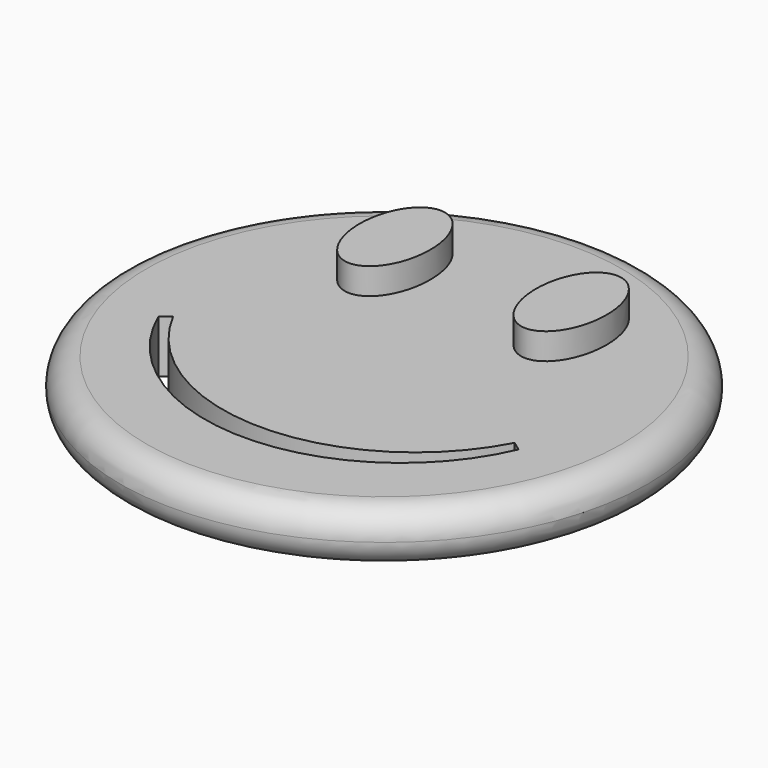
from build123d import *

# Parameters (mm, degrees)
F1_R     = 50
F3_DEPTH = 10
F4_DEPTH = 10
F5_DEPTH = 15
F6_R     = 4.99999


# Not quite as in the source:
# - a fillet or chamfer is up to 0.001 mm smaller than in the source, because OpenCascade refuses the exact size


with BuildPart() as f3:
    # F1 (on Top) → F3 (new body)
    with BuildSketch(Plane.XY):
        Circle(F1_R)
    extrude(amount=F3_DEPTH)

    # F2 (on Top) → F4 (cut, through all)
    with BuildSketch(Plane.XY):
        with BuildLine():
            ThreePointArc((-32.3443888766, -9.5336334546), (-33.1781101303, -10.2242371738), (-34.0725456744, -10.8341631392))
            ThreePointArc((-34.0725456744, -10.8341631392), (0.0457985584, -33.2293777169), (34.1692118563, -10.8418875925))
            Line((34.1692118563, -10.8418875925), (32.3708786214, -9.5576704707))
            ThreePointArc((32.3708786214, -9.5576704707), (0.0059751961, -29.1179251405), (-32.3443888766, -9.5336334546))
        make_face()
    extrude(amount=F4_DEPTH, mode=Mode.SUBTRACT)

    # F0 (on Top) → F5 (join)
    with BuildSketch(Plane.XY):
        with BuildLine():
            add(Edge.make_bspline(
                [(-16.6987832636, 12.6141887158), (-5.1069345829, 12.6141887158), (-10.9028589232, 28.8324337453), (-16.6987832636, 45.0506787747), (-22.4947076039, 28.8324337453), (-28.2906319443, 12.6141887158), (-16.6987832636, 12.6141887158)],
                knots=[0, 0, 0, 2.0943951024, 2.0943951024, 4.1887902048, 4.1887902048, 6.2831853072, 6.2831853072, 6.2831853072], degree=2, weights=[1, 0.5, 1, 0.5, 1, 0.5, 1]))
        make_face()
        with BuildLine():
            add(Edge.make_bspline(
                [(16.6987832636, 12.6141887158), (28.2906319443, 12.6141887158), (22.4947076039, 28.8324337453), (16.6987832636, 45.0506787747), (10.9028589232, 28.8324337453), (5.1069345829, 12.6141887158), (16.6987832636, 12.6141887158)],
                knots=[0, 0, 0, 2.0943951024, 2.0943951024, 4.1887902048, 4.1887902048, 6.2831853072, 6.2831853072, 6.2831853072], degree=2, weights=[1, 0.5, 1, 0.5, 1, 0.5, 1]))
        make_face()
    extrude(amount=F5_DEPTH)

    # F6 (radius 5 in the source; OpenCascade refuses exactly that, so slightly less here)
    f6_edges = [f3.edges().sort_by_distance(p)[0] for p in [
        (-50, 0, 10),
        (-50, 0, 0),
    ]]
    fillet(f6_edges, radius=F6_R)


solid = f3.part
